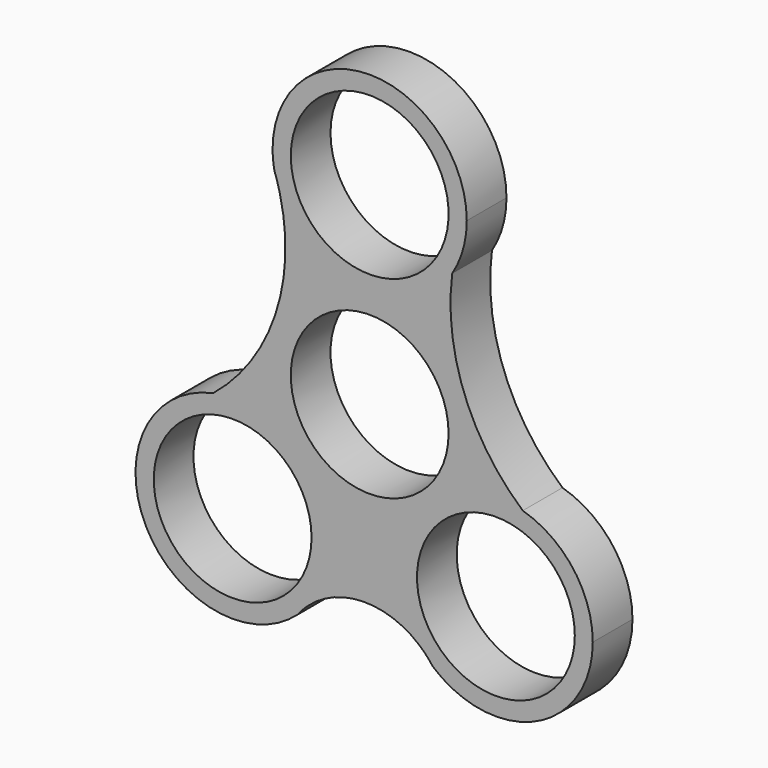
from build123d import *

# Parameters (mm, degrees)
F0_R         = 11.125
F1_DEPTH     = 7
F2_TEXT_SIZE = 5.6145120955
F3_DEPTH     = 7
F4_TEXT_SIZE = 6.9476046418
F5_DEPTH     = 7


# Not quite as in the source:
# - Text() gives the source's letters only with a copy of the font that has no kerning and outlines rounded to 1/6400 em; it was checked with that copy


with BuildPart() as f1:
    # F0 (on Front) → F1 (new body)
    with BuildSketch(Plane.XZ):
        with BuildLine():
            ThreePointArc((21.5884644556, -6.1726498392), (13.3315287594, 5.6903960682), (11.6399957989, 20.0447529515))
            ThreePointArc((11.6399957989, 20.0447529515), (-1.1299366923, 13.6071142972), (-12.6667741213, 22.0578982495))
            ThreePointArc((-12.6667741213, 22.0578982495), (-13.3254679122, 6.7616906408), (-22.0833336999, -5.7964792721))
            ThreePointArc((-22.0833336999, -5.7964792721), (-10.6656247325, -8.5963811827), (-5.6217310947, -19.2153578634))
            ThreePointArc((-5.6217310947, -19.2153578634), (-6.3889307767, -23.7356238038), (-8.6046040178, -27.7496232573))
            ThreePointArc((-8.6046040178, -27.7496232573), (-0.8863846152, -24.7802874171), (6.9092190223, -27.5400754536))
            ThreePointArc((6.9092190223, -27.5400754536), (6.5403231682, -11.5606738691), (21.5884644556, -6.1726498392))
        make_face()
        Circle(F0_R, mode=Mode.SUBTRACT)
        with BuildLine():
            Line((13.6895977745, 27.25), (11.125, 27.25))
            ThreePointArc((11.125, 27.25), (0, 16.125), (-11.125, 27.25))
            Line((-11.125, 27.25), (-13.6895977745, 27.25))
            ThreePointArc((-13.6895977745, 27.25), (-13.627830323, 25.9510281319), (-13.443085358, 24.6637781832))
            ThreePointArc((-13.443085358, 24.6637781832), (-13.0226063475, 23.3704675981), (-12.6667741213, 22.0578982495))
            ThreePointArc((-12.6667741213, 22.0578982495), (-1.1299366923, 13.6071142972), (11.6399957989, 20.0447529515))
            ThreePointArc((11.6399957989, 20.0447529515), (13.1672310645, 23.5044542024), (13.6895977745, 27.25))
        make_face()
        with BuildLine():
            ThreePointArc((-11.125, 27.25), (0, 38.375), (11.125, 27.25))
            Line((11.125, 27.25), (13.6895977745, 27.25))
            ThreePointArc((13.6895977745, 27.25), (0, 40.9395977745), (-13.6895977745, 27.25))
            Line((-13.6895977745, 27.25), (-11.125, 27.25))
        make_face()
        with BuildLine():
            ThreePointArc((31.4567178404, -19.2947368677), (28.7143466045, -11.0854190999), (21.5884644556, -6.1726498392))
            ThreePointArc((21.5884644556, -6.1726498392), (6.5403231682, -11.5606738691), (6.9092190223, -27.5400754536))
            ThreePointArc((6.9092190223, -27.5400754536), (7.9696267547, -28.5379831954), (8.9006293155, -29.6575896672))
            ThreePointArc((8.9006293155, -29.6575896672), (23.500285506, -31.7060809497), (31.4567178404, -19.2947368677))
        make_face()
        with Locations((17.7981917398, -19.2947368677)):
            Circle(F0_R, mode=Mode.SUBTRACT)
        with BuildLine():
            ThreePointArc((-5.6217310947, -19.2153578634), (-10.6656247325, -8.5963811827), (-22.0833336999, -5.7964792721))
            ThreePointArc((-22.0833336999, -5.7964792721), (-31.5481020918, -25.3967966847), (-10.152487057, -29.3945386312))
            ThreePointArc((-10.152487057, -29.3945386312), (-9.4175428443, -28.5353840595), (-8.6046040178, -27.7496232573))
            ThreePointArc((-8.6046040178, -27.7496232573), (-6.3889307767, -23.7356238038), (-5.6217310947, -19.2153578634))
        make_face()
        with Locations((-19.321814671, -19.2153578634)):
            Circle(F0_R, mode=Mode.SUBTRACT)
    extrude(amount=F1_DEPTH)

    # F2 (on Front) → F3 (join)
    with BuildSketch(Plane.XZ):
        with Locations((12.0921619236, -5.9908139519)):
            Text('Lp', F2_TEXT_SIZE, font='Open Sans', text_align=(TextAlign.LEFT, TextAlign.BOTTOM))
    extrude(amount=F3_DEPTH)

    # F4 (on Front) → F5 (join)
    with BuildSketch(Plane.XZ):
        with Locations((10.5974478647, -6.5792017849)):
            Text('Lp', F4_TEXT_SIZE, font='Open Sans', text_align=(TextAlign.LEFT, TextAlign.BOTTOM))
    extrude(amount=F5_DEPTH)


solid = f1.part
